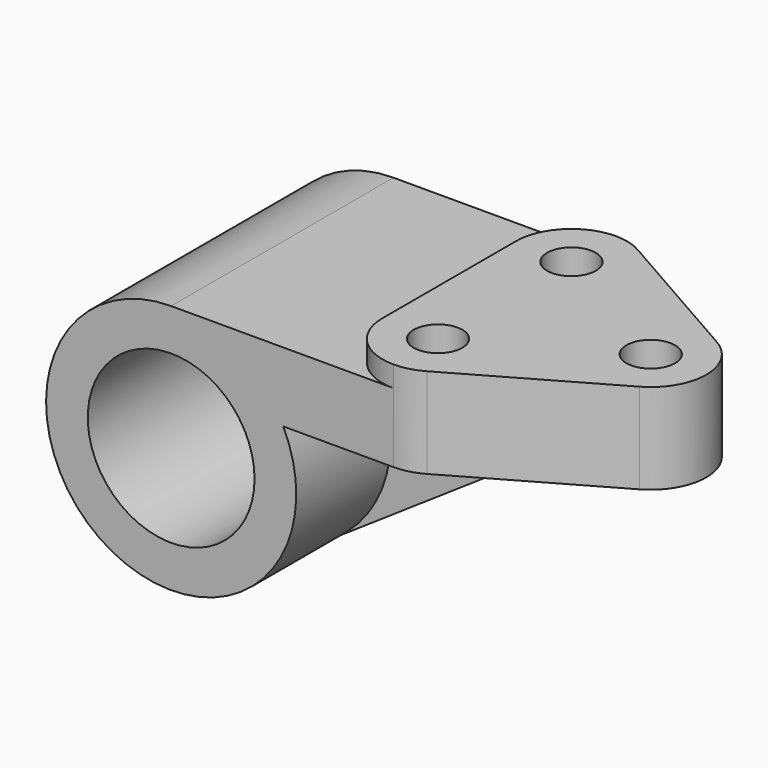
from build123d import *

# Parameters (mm, degrees)
F0_R     = 19.05
F1_DEPTH = 31.75
F2_R     = 5.5626
F3_DEPTH = 20.6502
F4_DEPTH = 57.151
F6_DEPTH = 4.7625


with BuildPart() as f1:
    # F0 (on Front) → F1 (new body, symmetric)
    with BuildSketch(Plane.XZ):
        with BuildLine():
            Line((50.8, 28.575), (0, 28.575))
            ThreePointArc((0, 28.575), (-15.0603473566, -24.2840804335), (25.5976683508, 12.7))
            Line((25.5976683508, 12.7), (50.8, 12.7))
            Line((50.8, 12.7), (50.8, 28.575))
        make_face()
        Circle(F0_R, mode=Mode.SUBTRACT)
    extrude(amount=F1_DEPTH, both=True)

    # F2 (on face) → F3 (join)
    with BuildSketch(Plane(origin=(0, 0, 12.7), x_dir=(1, 0, 0), z_dir=(0, 0, -1))):
        with BuildLine():
            Line((50.8, 24.6126), (50.8, 31.75))
            ThreePointArc((50.8, 31.75), (41.8197438789, 28.0302561211), (38.1, 19.05))
            Line((38.1, 19.05), (38.1, -19.05))
            ThreePointArc((38.1, -19.05), (41.8197438789, -28.0302561211), (50.8, -31.75))
            Line((50.8, -31.75), (50.8, -24.6126))
            ThreePointArc((50.8, -24.6126), (45.2374, -19.05), (50.8, -13.4874))
            Line((50.8, -13.4874), (50.8, 13.4874))
            ThreePointArc((50.8, 13.4874), (45.2374, 19.05), (50.8, 24.6126))
        make_face()
        with BuildLine():
            Line((90.4493554441, 11.0277214642), (57.0991554441, 30.0777214642))
            ThreePointArc((57.0991554441, 30.0777214642), (54.0586759125, 31.3248128824), (50.8, 31.75))
            Line((50.8, 31.75), (50.8, 24.6126))
            ThreePointArc((50.8, 24.6126), (54.733352181, 22.983352181), (56.3626, 19.05))
            ThreePointArc((56.3626, 19.05), (54.733352181, 15.116647819), (50.8, 13.4874))
            Line((50.8, 13.4874), (50.8, -13.4874))
            ThreePointArc((50.8, -13.4874), (54.733352181, -15.116647819), (56.3626, -19.05))
            ThreePointArc((56.3626, -19.05), (54.733352181, -22.983352181), (50.8, -24.6126))
            Line((50.8, -24.6126), (50.8, -31.75))
            ThreePointArc((50.8, -31.75), (54.0586759125, -31.3248128824), (57.0991554441, -30.0777214642))
            Line((57.0991554441, -30.0777214642), (90.4493554441, -11.0277214642))
            ThreePointArc((90.4493554441, -11.0277214642), (96.8502, 0), (90.4493554441, 11.0277214642))
        make_face()
        with Locations((84.1502, 0)):
            Circle(F2_R, mode=Mode.SUBTRACT)
    extrude(amount=-F3_DEPTH)

    # F4 (cut, through all): faces of the model
    f4_faces = [f1.faces().sort_by_distance(p)[0] for p in [
        (48.4391592362, 19.05, 28.575),
        (48.4391592362, -19.05, 28.575),
    ]]
    extrude(f4_faces, amount=-F4_DEPTH, mode=Mode.SUBTRACT)

    # F5 (on Front) → F6 (join, symmetric)
    with BuildSketch(Plane.XZ):
        with BuildLine():
            ThreePointArc((25.5976683508, 12.7), (27.6286795727, -7.2929205446), (15.9950252975, -23.6788891364))
            Line((15.9950252975, -23.6788891364), (69.85, 12.7))
            Line((69.85, 12.7), (25.5976683508, 12.7))
        make_face()
    extrude(amount=F6_DEPTH, both=True)


solid = f1.part
